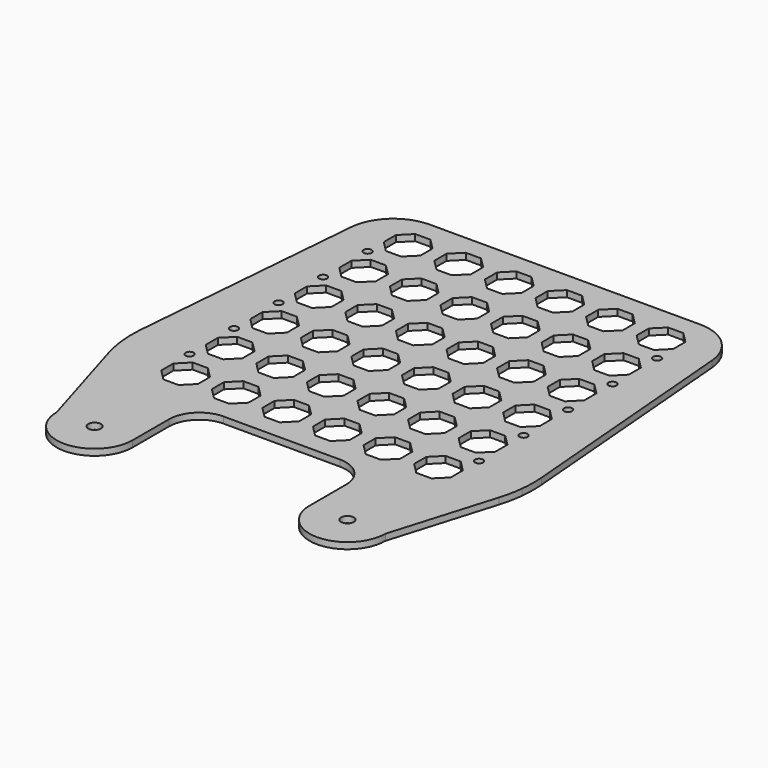
from build123d import *

# Parameters (mm, degrees)
F1_DEPTH = 3.175
F2_R     = 2.032
F3_DEPTH = 3.176


with BuildPart() as f1:
    # F0 (on Top) → F1 (new body)
    with BuildSketch(Plane.XY):
        with BuildLine():
            Line((67.8657623274, 152.4), (-67.8657623274, 152.4))
            ThreePointArc((-67.8657623274, 152.4), (-83.3444852456, 146.3622690747), (-90.6467983609, 131.4384196695))
            Line((-90.6467983609, 131.4384196695), (-100.6005854186, 11.9929749763))
            ThreePointArc((-100.6005854186, 11.9929749763), (-100.8157754748, 5.993241191), (-100.463394598, 0))
            Line((-100.463394598, 0), (100.463394598, 0))
            ThreePointArc((100.463394598, 0), (100.8157754748, 5.993241191), (100.6005854186, 11.9929749763))
            Line((100.6005854186, 11.9929749763), (90.6467983609, 131.4384196695))
            ThreePointArc((90.6467983609, 131.4384196695), (83.3444852456, 146.3622690747), (67.8657623274, 152.4))
        make_face()
        with BuildLine():
            Line((100.463394598, 0), (-100.463394598, 0))
            ThreePointArc((-100.463394598, 0), (-99.5700314301, -5.817352147), (-98.1418988816, -11.5270037279))
            Line((-98.1418988816, -11.5270037279), (-82.55, -63.5))
            ThreePointArc((-82.55, -63.5), (-63.5, -44.45), (-44.45, -63.5))
            Line((-44.45, -63.5), (-44.45, -40.64))
            ThreePointArc((-44.45, -40.64), (-39.9863073453, -29.8636926547), (-29.21, -25.4))
            Line((-29.21, -25.4), (29.21, -25.4))
            ThreePointArc((29.21, -25.4), (39.9863073453, -29.8636926547), (44.45, -40.64))
            Line((44.45, -40.64), (44.45, -63.5))
            ThreePointArc((44.45, -63.5), (63.5, -44.45), (82.55, -63.5))
            Line((82.55, -63.5), (98.1418988816, -11.5270037279))
            ThreePointArc((98.1418988816, -11.5270037279), (99.5700314301, -5.817352147), (100.463394598, 0))
        make_face()
        with BuildLine():
            ThreePointArc((-44.45, -63.5), (-63.5, -44.45), (-82.55, -63.5))
            Line((-82.55, -63.5), (-66.675, -63.5))
            ThreePointArc((-66.675, -63.5), (-63.5, -60.325), (-60.325, -63.5))
            Line((-60.325, -63.5), (-44.45, -63.5))
        make_face()
        with BuildLine():
            Line((-66.675, -63.5), (-82.55, -63.5))
            ThreePointArc((-82.55, -63.5), (-63.5, -82.55), (-44.45, -63.5))
            Line((-44.45, -63.5), (-60.325, -63.5))
            ThreePointArc((-60.325, -63.5), (-63.5, -66.675), (-66.675, -63.5))
        make_face()
        with BuildLine():
            ThreePointArc((44.45, -63.5), (63.5, -82.55), (82.55, -63.5))
            Line((82.55, -63.5), (66.675, -63.5))
            ThreePointArc((66.675, -63.5), (63.5, -66.675), (60.325, -63.5))
            Line((60.325, -63.5), (44.45, -63.5))
        make_face()
        with BuildLine():
            Line((66.675, -63.5), (82.55, -63.5))
            ThreePointArc((82.55, -63.5), (63.5, -44.45), (44.45, -63.5))
            Line((44.45, -63.5), (60.325, -63.5))
            ThreePointArc((60.325, -63.5), (63.5, -60.325), (66.675, -63.5))
        make_face()
    extrude(amount=F1_DEPTH)

    # F2 (on face) → F3 (cut, through all)
    with BuildSketch(Plane.XY.offset(3.175)):
        Polygon((-59.69, 124.1518463274), (-54.3018463274, 129.54), (-54.3018463274, 137.16), (-59.69, 142.5481536726), (-67.31, 142.5481536726), (-72.6981536726, 137.16), (-72.6981536726, 129.54), (-67.31, 124.1518463274), align=None)
        Polygon((-72.6981536726, 101.6), (-67.31, 96.2118463274), (-59.69, 96.2118463274), (-54.3018463274, 101.6), (-54.3018463274, 109.22), (-59.69, 114.6081536726), (-67.31, 114.6081536726), (-72.6981536726, 109.22), align=None)
        Polygon((-72.6981536726, 73.66), (-67.31, 68.2718463274), (-59.69, 68.2718463274), (-54.3018463274, 73.66), (-54.3018463274, 81.28), (-59.69, 86.6681536726), (-67.31, 86.6681536726), (-72.6981536726, 81.28), align=None)
        Polygon((-72.6981536726, 45.72), (-67.31, 40.3318463274), (-59.69, 40.3318463274), (-54.3018463274, 45.72), (-54.3018463274, 53.34), (-59.69, 58.7281536726), (-67.31, 58.7281536726), (-72.6981536726, 53.34), align=None)
        Polygon((-72.6981536726, 17.78), (-67.31, 12.3918463274), (-59.69, 12.3918463274), (-54.3018463274, 17.78), (-54.3018463274, 25.4), (-59.69, 30.7881536726), (-67.31, 30.7881536726), (-72.6981536726, 25.4), align=None)
        Polygon((-72.6981536726, -10.16), (-67.31, -15.5481536726), (-59.69, -15.5481536726), (-54.3018463274, -10.16), (-54.3018463274, -2.54), (-59.69, 2.8481536726), (-67.31, 2.8481536726), (-72.6981536726, -2.54), align=None)
        Polygon((-47.2981536726, 129.54), (-41.91, 124.1518463274), (-34.29, 124.1518463274), (-28.9018463274, 129.54), (-28.9018463274, 137.16), (-34.29, 142.5481536726), (-41.91, 142.5481536726), (-47.2981536726, 137.16), align=None)
        Polygon((-47.2981536726, 101.6), (-41.91, 96.2118463274), (-34.29, 96.2118463274), (-28.9018463274, 101.6), (-28.9018463274, 109.22), (-34.29, 114.6081536726), (-41.91, 114.6081536726), (-47.2981536726, 109.22), align=None)
        Polygon((-47.2981536726, 73.66), (-41.91, 68.2718463274), (-34.29, 68.2718463274), (-28.9018463274, 73.66), (-28.9018463274, 81.28), (-34.29, 86.6681536726), (-41.91, 86.6681536726), (-47.2981536726, 81.28), align=None)
        Polygon((-47.2981536726, 45.72), (-41.91, 40.3318463274), (-34.29, 40.3318463274), (-28.9018463274, 45.72), (-28.9018463274, 53.34), (-34.29, 58.7281536726), (-41.91, 58.7281536726), (-47.2981536726, 53.34), align=None)
        Polygon((-47.2981536726, 17.78), (-41.91, 12.3918463274), (-34.29, 12.3918463274), (-28.9018463274, 17.78), (-28.9018463274, 25.4), (-34.29, 30.7881536726), (-41.91, 30.7881536726), (-47.2981536726, 25.4), align=None)
        Polygon((-47.2981536726, -10.16), (-41.91, -15.5481536726), (-34.29, -15.5481536726), (-28.9018463274, -10.16), (-28.9018463274, -2.54), (-34.29, 2.8481536726), (-41.91, 2.8481536726), (-47.2981536726, -2.54), align=None)
        Polygon((-21.8981536726, 129.54), (-16.51, 124.1518463274), (-8.89, 124.1518463274), (-3.5018463274, 129.54), (-3.5018463274, 137.16), (-8.89, 142.5481536726), (-16.51, 142.5481536726), (-21.8981536726, 137.16), align=None)
        Polygon((-21.8981536726, 101.6), (-16.51, 96.2118463274), (-8.89, 96.2118463274), (-3.5018463274, 101.6), (-3.5018463274, 109.22), (-8.89, 114.6081536726), (-16.51, 114.6081536726), (-21.8981536726, 109.22), align=None)
        Polygon((-21.8981536726, 73.66), (-16.51, 68.2718463274), (-8.89, 68.2718463274), (-3.5018463274, 73.66), (-3.5018463274, 81.28), (-8.89, 86.6681536726), (-16.51, 86.6681536726), (-21.8981536726, 81.28), align=None)
        Polygon((-21.8981536726, 45.72), (-16.51, 40.3318463274), (-8.89, 40.3318463274), (-3.5018463274, 45.72), (-3.5018463274, 53.34), (-8.89, 58.7281536726), (-16.51, 58.7281536726), (-21.8981536726, 53.34), align=None)
        Polygon((-21.8981536726, 17.78), (-16.51, 12.3918463274), (-8.89, 12.3918463274), (-3.5018463274, 17.78), (-3.5018463274, 25.4), (-8.89, 30.7881536726), (-16.51, 30.7881536726), (-21.8981536726, 25.4), align=None)
        Polygon((-21.8981536726, -10.16), (-16.51, -15.5481536726), (-8.89, -15.5481536726), (-3.5018463274, -10.16), (-3.5018463274, -2.54), (-8.89, 2.8481536726), (-16.51, 2.8481536726), (-21.8981536726, -2.54), align=None)
        Polygon((72.6981536726, 137.16), (67.31, 142.5481536726), (59.69, 142.5481536726), (54.3018463274, 137.16), (54.3018463274, 129.54), (59.69, 124.1518463274), (67.31, 124.1518463274), (72.6981536726, 129.54), align=None)
        Polygon((59.69, 96.2118463274), (67.31, 96.2118463274), (72.6981536726, 101.6), (72.6981536726, 109.22), (67.31, 114.6081536726), (59.69, 114.6081536726), (54.3018463274, 109.22), (54.3018463274, 101.6), align=None)
        Polygon((28.9018463274, 129.54), (34.29, 124.1518463274), (41.91, 124.1518463274), (47.2981536726, 129.54), (47.2981536726, 137.16), (41.91, 142.5481536726), (34.29, 142.5481536726), (28.9018463274, 137.16), align=None)
        Polygon((72.6981536726, 53.34), (67.31, 58.7281536726), (59.69, 58.7281536726), (54.3018463274, 53.34), (54.3018463274, 45.72), (59.69, 40.3318463274), (67.31, 40.3318463274), (72.6981536726, 45.72), align=None)
        Polygon((47.2981536726, -2.54), (41.91, 2.8481536726), (34.29, 2.8481536726), (28.9018463274, -2.54), (28.9018463274, -10.16), (34.29, -15.5481536726), (41.91, -15.5481536726), (47.2981536726, -10.16), align=None)
        Polygon((47.2981536726, 53.34), (41.91, 58.7281536726), (34.29, 58.7281536726), (28.9018463274, 53.34), (28.9018463274, 45.72), (34.29, 40.3318463274), (41.91, 40.3318463274), (47.2981536726, 45.72), align=None)
        Polygon((47.2981536726, 109.22), (41.91, 114.6081536726), (34.29, 114.6081536726), (28.9018463274, 109.22), (28.9018463274, 101.6), (34.29, 96.2118463274), (41.91, 96.2118463274), (47.2981536726, 101.6), align=None)
        Polygon((72.6981536726, -2.54), (67.31, 2.8481536726), (59.69, 2.8481536726), (54.3018463274, -2.54), (54.3018463274, -10.16), (59.69, -15.5481536726), (67.31, -15.5481536726), (72.6981536726, -10.16), align=None)
        Polygon((21.8981536726, -2.54), (16.51, 2.8481536726), (8.89, 2.8481536726), (3.5018463274, -2.54), (3.5018463274, -10.16), (8.89, -15.5481536726), (16.51, -15.5481536726), (21.8981536726, -10.16), align=None)
        Polygon((21.8981536726, 53.34), (16.51, 58.7281536726), (8.89, 58.7281536726), (3.5018463274, 53.34), (3.5018463274, 45.72), (8.89, 40.3318463274), (16.51, 40.3318463274), (21.8981536726, 45.72), align=None)
        Polygon((21.8981536726, 109.22), (16.51, 114.6081536726), (8.89, 114.6081536726), (3.5018463274, 109.22), (3.5018463274, 101.6), (8.89, 96.2118463274), (16.51, 96.2118463274), (21.8981536726, 101.6), align=None)
        Polygon((59.69, 12.3918463274), (67.31, 12.3918463274), (72.6981536726, 17.78), (72.6981536726, 25.4), (67.31, 30.7881536726), (59.69, 30.7881536726), (54.3018463274, 25.4), (54.3018463274, 17.78), align=None)
        Polygon((59.69, 68.2718463274), (67.31, 68.2718463274), (72.6981536726, 73.66), (72.6981536726, 81.28), (67.31, 86.6681536726), (59.69, 86.6681536726), (54.3018463274, 81.28), (54.3018463274, 73.66), align=None)
        Polygon((8.89, 124.1518463274), (16.51, 124.1518463274), (21.8981536726, 129.54), (21.8981536726, 137.16), (16.51, 142.5481536726), (8.89, 142.5481536726), (3.5018463274, 137.16), (3.5018463274, 129.54), align=None)
        Polygon((34.29, 12.3918463274), (41.91, 12.3918463274), (47.2981536726, 17.78), (47.2981536726, 25.4), (41.91, 30.7881536726), (34.29, 30.7881536726), (28.9018463274, 25.4), (28.9018463274, 17.78), align=None)
        Polygon((34.29, 68.2718463274), (41.91, 68.2718463274), (47.2981536726, 73.66), (47.2981536726, 81.28), (41.91, 86.6681536726), (34.29, 86.6681536726), (28.9018463274, 81.28), (28.9018463274, 73.66), align=None)
        Polygon((8.89, 12.3918463274), (16.51, 12.3918463274), (21.8981536726, 17.78), (21.8981536726, 25.4), (16.51, 30.7881536726), (8.89, 30.7881536726), (3.5018463274, 25.4), (3.5018463274, 17.78), align=None)
        Polygon((8.89, 68.2718463274), (16.51, 68.2718463274), (21.8981536726, 73.66), (21.8981536726, 81.28), (16.51, 86.6681536726), (8.89, 86.6681536726), (3.5018463274, 81.28), (3.5018463274, 73.66), align=None)
        with Locations((72.6981536726, 63.5)):
            Circle(F2_R)
        with Locations((72.6981536726, 35.56)):
            Circle(F2_R)
        with Locations((72.6981536726, 7.62)):
            Circle(F2_R)
        with Locations((72.6981536726, 119.38)):
            Circle(F2_R)
        with Locations((72.6981536726, 91.44)):
            Circle(F2_R)
        with Locations((-72.6981536726, 119.38)):
            Circle(F2_R)
        with Locations((-72.6981536726, 91.44)):
            Circle(F2_R)
        with Locations((-72.6981536726, 63.5)):
            Circle(F2_R)
        with Locations((-72.6981536726, 35.56)):
            Circle(F2_R)
        with Locations((-72.6981536726, 7.62)):
            Circle(F2_R)
    extrude(amount=-F3_DEPTH, mode=Mode.SUBTRACT)


solid = f1.part
